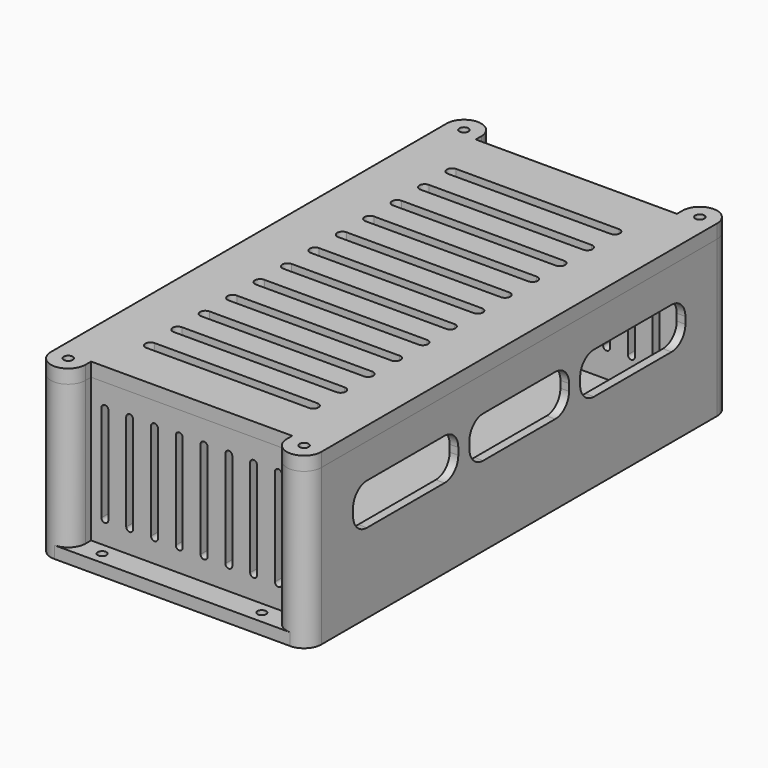
from build123d import *

# Parameters (mm, degrees)
F0_W      = 78.13
F0_H      = 138.9
F0_W_2    = 71.13
F0_H_2    = 131.9
F1_DEPTH  = 25
F2_W      = 71.13
F2_H      = 131.9
F3_DEPTH  = 2
F4_R      = 1.8
F5_DEPTH  = 6
F6_DEPTH  = 15
F7_DEPTH  = 5
F9_DEPTH  = 25
F11_DEPTH = 3.5
F12_W     = 73.13
F12_H     = 133.9
F12_W_2   = 71.13
F12_H_2   = 131.9
F13_DEPTH = 37
F14_W     = 56.34
F14_H     = 1
F14_W_2   = 1
F14_H_2   = 116.795
F14_H_3   = 107.2624295342
F15_DEPTH = 6
F17_DEPTH = 45
F19_DEPTH = 4
F20_W     = 72.53
F20_H     = 133.3
F21_DEPTH = 2
F23_DEPTH = 10
F24_R     = 1.3
F25_DEPTH = 20
F26_R     = 1.3
F27_DEPTH = 15
F28_W     = 68.13
F28_H     = 7
F29_DEPTH = 3.5
F30_R     = 1.25
F31_DEPTH = 25
F32_R     = 1.25
F33_DEPTH = 25
F35_DEPTH = 213


with BuildPart() as f1:
    # F0 (on Top) → F1 (new body)
    with BuildSketch(Plane.XY):
        with Locations((-1.6999974132, -1.6999974132)):
            Rectangle(F0_W, F0_H)
        with Locations((-1.6999974132, -1.6999974132)):
            Rectangle(F0_W_2, F0_H_2, mode=Mode.SUBTRACT)
    extrude(amount=F1_DEPTH)

    # F2 (on face) → F3 (join)
    with BuildSketch(Plane(origin=(0, 0, 0), x_dir=(1, 0, 0), z_dir=(0, 0, -1))):
        with Locations((-1.6999974132, 1.6999974132)):
            Rectangle(F2_W, F2_H)
    extrude(amount=-F3_DEPTH)

    # F4 (on face) → F5 (join)
    with BuildSketch(Plane.XY.offset(2)):
        with BuildLine():
            ThreePointArc((30.1700025868, -59.9299974132), (27.8294791411, -60.8994739674), (26.8600025868, -63.2399974132))
            Line((26.8600025868, -63.2399974132), (26.8600025868, -67.1499974132))
            Line((26.8600025868, -67.1499974132), (26.8600025868, -67.6499974132))
            Line((26.8600025868, -67.6499974132), (33.8650025868, -67.6499974132))
            Line((33.8650025868, -67.6499974132), (33.8650025868, -59.9299974132))
            Line((33.8650025868, -59.9299974132), (33.3000025868, -59.9299974132))
            Line((33.3000025868, -59.9299974132), (30.1700025868, -59.9299974132))
        make_face()
        with Locations((30.1700025868, -63.2399974132)):
            Circle(F4_R, mode=Mode.SUBTRACT)
        with BuildLine():
            ThreePointArc((-29.4799974132, -63.6399974132), (-30.566631255, -61.016631255), (-33.1899974132, -59.9299974132))
            Line((-33.1899974132, -59.9299974132), (-36.6999974132, -59.9299974132))
            Line((-36.6999974132, -59.9299974132), (-37.2649974132, -59.9299974132))
            Line((-37.2649974132, -59.9299974132), (-37.2649974132, -67.6499974132))
            Line((-37.2649974132, -67.6499974132), (-29.4799974132, -67.6499974132))
            Line((-29.4799974132, -67.6499974132), (-29.4799974132, -67.1499974132))
            Line((-29.4799974132, -67.1499974132), (-29.4799974132, -63.6399974132))
        make_face()
        with Locations((-33.1899974132, -63.6399974132)):
            Circle(F4_R, mode=Mode.SUBTRACT)
        with BuildLine():
            Line((-36.6999974132, 47.3750025868), (-33.6899974132, 47.3750025868))
            ThreePointArc((-33.6899974132, 47.3750025868), (-30.0649974132, 51.0000025868), (-33.6899974132, 54.6250025868))
            Line((-33.6899974132, 54.6250025868), (-36.6999974132, 54.6250025868))
            Line((-36.6999974132, 54.6250025868), (-37.2649974132, 54.6250025868))
            Line((-37.2649974132, 54.6250025868), (-37.2649974132, 47.3750025868))
            Line((-37.2649974132, 47.3750025868), (-36.6999974132, 47.3750025868))
        make_face()
        with Locations((-33.6899974132, 51.0000025868)):
            Circle(F4_R, mode=Mode.SUBTRACT)
        with BuildLine():
            Line((26.4150025868, 63.7500025868), (26.4150025868, 60.4900025868))
            ThreePointArc((26.4150025868, 60.4900025868), (27.476740505, 57.926740505), (30.0400025868, 56.8650025868))
            Line((30.0400025868, 56.8650025868), (33.8650025868, 56.8650025868))
            Line((33.8650025868, 56.8650025868), (33.8650025868, 64.2500025868))
            Line((33.8650025868, 64.2500025868), (26.4150025868, 64.2500025868))
            Line((26.4150025868, 64.2500025868), (26.4150025868, 63.7500025868))
        make_face()
        with BuildLine():
            ThreePointArc((30.0400025868, 58.6900025868), (28.7672103807, 61.762794793), (31.8400025868, 60.4900025868))
            ThreePointArc((31.8400025868, 60.4900025868), (31.312794793, 59.2172103807), (30.0400025868, 58.6900025868))
        make_face(mode=Mode.SUBTRACT)
    extrude(amount=F5_DEPTH)

    # F6 (add): a face of the model
    f6_faces = [f1.faces().sort_by_distance(p)[0] for p in [
        (35.7713430592, -1.6999974132, 25),
    ]]
    extrude(f6_faces, amount=F6_DEPTH)

    # F7 (add): a face of the model
    f7_faces = [f1.faces().sort_by_distance(p)[0] for p in [
        (35.7713430592, -1.6999974132, 40),
    ]]
    extrude(f7_faces, amount=F7_DEPTH)

    # F8 (on face) → F9 (cut)
    with BuildSketch(Plane.YZ.offset(37.3650025868)):
        with BuildLine():
            Line((11.3000025868, 35), (-1.6999974132, 35))
            Line((-1.6999974132, 35), (-14.6999974132, 35))
            ThreePointArc((-14.6999974132, 35), (-18.2355313191, 33.5355339059), (-19.6999974132, 30))
            Line((-19.6999974132, 30), (-19.6999974132, 28))
            ThreePointArc((-19.6999974132, 28), (-18.2355313191, 24.4644660941), (-14.6999974132, 23))
            Line((-14.6999974132, 23), (11.3000025868, 23))
            ThreePointArc((11.3000025868, 23), (14.8355364928, 24.4644660941), (16.3000025868, 28))
            Line((16.3000025868, 28), (16.3000025868, 30))
            ThreePointArc((16.3000025868, 30), (14.8355364928, 33.5355339059), (11.3000025868, 35))
        make_face()
        with BuildLine():
            Line((58.3000025868, 28), (58.3000025868, 30))
            ThreePointArc((58.3000025868, 30), (56.8355364928, 33.5355339059), (53.3000025868, 35))
            Line((53.3000025868, 35), (25.3000025868, 35))
            ThreePointArc((25.3000025868, 35), (21.7644686809, 33.5355339059), (20.3000025868, 30))
            Line((20.3000025868, 30), (20.3000025868, 28))
            ThreePointArc((20.3000025868, 28), (21.7644686809, 24.4644660941), (25.3000025868, 23))
            Line((25.3000025868, 23), (53.3000025868, 23))
            ThreePointArc((53.3000025868, 23), (56.8355364928, 24.4644660941), (58.3000025868, 28))
        make_face()
        with BuildLine():
            Line((-61.6999974132, 30), (-61.6999974132, 28))
            ThreePointArc((-61.6999974132, 28), (-60.2355313191, 24.4644660941), (-56.6999974132, 23))
            Line((-56.6999974132, 23), (-28.6999974132, 23))
            ThreePointArc((-28.6999974132, 23), (-25.1644635072, 24.4644660941), (-23.6999974132, 28))
            Line((-23.6999974132, 28), (-23.6999974132, 30))
            ThreePointArc((-23.6999974132, 30), (-25.1644635072, 33.5355339059), (-28.6999974132, 35))
            Line((-28.6999974132, 35), (-56.6999974132, 35))
            ThreePointArc((-56.6999974132, 35), (-60.2355313191, 33.5355339059), (-61.6999974132, 30))
        make_face()
    extrude(amount=-F9_DEPTH, mode=Mode.SUBTRACT)

    # F10 (on face) → F11 (cut, through all)
    with BuildSketch(Plane(origin=(-40.7649974132, 0, 0), x_dir=(0, -1, 0), z_dir=(-1, 0, 0))):
        with BuildLine():
            ThreePointArc((-59.6591697992, 39), (-60.0000025868, 39.03351143), (-60.3408353745, 39))
            Line((-60.3408353745, 39), (-59.6591697992, 39))
        make_face()
        with BuildLine():
            Line((-59.6591697992, 39), (-60.3408353745, 39))
            ThreePointArc((-60.3408353745, 39), (-61.3525848169, 38.3939263573), (-61.7500025868, 37.28351143))
            Line((-61.7500025868, 37.28351143), (-61.7500025868, 7.75))
            ThreePointArc((-61.7500025868, 7.75), (-60.0000025868, 6), (-58.2500025868, 7.75))
            Line((-58.2500025868, 7.75), (-58.2500025868, 37.28351143))
            ThreePointArc((-58.2500025868, 37.28351143), (-58.6474203567, 38.3939263573), (-59.6591697992, 39))
        make_face()
        with BuildLine():
            ThreePointArc((-46.6408353745, 39), (-47.6525848169, 38.3939263573), (-48.0500025868, 37.28351143))
            Line((-48.0500025868, 37.28351143), (-48.0500025868, 7.75))
            ThreePointArc((-48.0500025868, 7.75), (-46.3000025868, 6), (-44.5500025868, 7.75))
            Line((-44.5500025868, 7.75), (-44.5500025868, 37.28351143))
            ThreePointArc((-44.5500025868, 37.28351143), (-44.9474203567, 38.3939263573), (-45.9591697992, 39))
            Line((-45.9591697992, 39), (-46.6408353745, 39))
        make_face()
        with BuildLine():
            ThreePointArc((-45.9591697992, 39), (-46.3000025868, 39.03351143), (-46.6408353745, 39))
            Line((-46.6408353745, 39), (-45.9591697992, 39))
        make_face()
        with BuildLine():
            ThreePointArc((-32.9408353745, 39), (-33.9525848169, 38.3939263573), (-34.3500025868, 37.28351143))
            Line((-34.3500025868, 37.28351143), (-34.3500025868, 7.75))
            ThreePointArc((-34.3500025868, 7.75), (-32.6000025868, 6), (-30.8500025868, 7.75))
            Line((-30.8500025868, 7.75), (-30.8500025868, 37.28351143))
            ThreePointArc((-30.8500025868, 37.28351143), (-31.2474203567, 38.3939263573), (-32.2591697992, 39))
            Line((-32.2591697992, 39), (-32.9408353745, 39))
        make_face()
        with BuildLine():
            ThreePointArc((-32.2591697992, 39), (-32.6000025868, 39.03351143), (-32.9408353745, 39))
            Line((-32.9408353745, 39), (-32.2591697992, 39))
        make_face()
        with BuildLine():
            ThreePointArc((-19.2408353745, 39), (-20.2525848169, 38.3939263573), (-20.6500025868, 37.28351143))
            Line((-20.6500025868, 37.28351143), (-20.6500025868, 7.75))
            ThreePointArc((-20.6500025868, 7.75), (-18.9000025868, 6), (-17.1500025868, 7.75))
            Line((-17.1500025868, 7.75), (-17.1500025868, 37.28351143))
            ThreePointArc((-17.1500025868, 37.28351143), (-17.5474203567, 38.3939263573), (-18.5591697992, 39))
            Line((-18.5591697992, 39), (-19.2408353745, 39))
        make_face()
        with BuildLine():
            ThreePointArc((-18.5591697992, 39), (-18.9000025868, 39.03351143), (-19.2408353745, 39))
            Line((-19.2408353745, 39), (-18.5591697992, 39))
        make_face()
        with BuildLine():
            ThreePointArc((-5.5408353745, 39), (-6.5525848169, 38.3939263573), (-6.9500025868, 37.28351143))
            Line((-6.9500025868, 37.28351143), (-6.9500025868, 7.75))
            ThreePointArc((-6.9500025868, 7.75), (-5.2000025868, 6), (-3.4500025868, 7.75))
            Line((-3.4500025868, 7.75), (-3.4500025868, 37.28351143))
            ThreePointArc((-3.4500025868, 37.28351143), (-3.8474203567, 38.3939263573), (-4.8591697992, 39))
            Line((-4.8591697992, 39), (-5.5408353745, 39))
        make_face()
        with BuildLine():
            ThreePointArc((-4.8591697992, 39), (-5.2000025868, 39.03351143), (-5.5408353745, 39))
            Line((-5.5408353745, 39), (-4.8591697992, 39))
        make_face()
        with BuildLine():
            ThreePointArc((8.1591646255, 39), (7.1474151831, 38.3939263573), (6.7499974132, 37.28351143))
            Line((6.7499974132, 37.28351143), (6.7499974132, 7.75))
            ThreePointArc((6.7499974132, 7.75), (8.4999974132, 6), (10.2499974132, 7.75))
            Line((10.2499974132, 7.75), (10.2499974132, 37.28351143))
            ThreePointArc((10.2499974132, 37.28351143), (9.8525796433, 38.3939263573), (8.8408302008, 39))
            Line((8.8408302008, 39), (8.1591646255, 39))
        make_face()
        with BuildLine():
            ThreePointArc((8.8408302008, 39), (8.4999974132, 39.03351143), (8.1591646255, 39))
            Line((8.1591646255, 39), (8.8408302008, 39))
        make_face()
        with BuildLine():
            ThreePointArc((21.8591646255, 39), (20.8474151831, 38.3939263573), (20.4499974132, 37.28351143))
            Line((20.4499974132, 37.28351143), (20.4499974132, 7.75))
            ThreePointArc((20.4499974132, 7.75), (22.1999974132, 6), (23.9499974132, 7.75))
            Line((23.9499974132, 7.75), (23.9499974132, 37.28351143))
            ThreePointArc((23.9499974132, 37.28351143), (23.5525796433, 38.3939263573), (22.5408302008, 39))
            Line((22.5408302008, 39), (21.8591646255, 39))
        make_face()
        with BuildLine():
            ThreePointArc((22.5408302008, 39), (22.1999974132, 39.03351143), (21.8591646255, 39))
            Line((21.8591646255, 39), (22.5408302008, 39))
        make_face()
        with BuildLine():
            ThreePointArc((35.5591646255, 39), (34.5474151831, 38.3939263573), (34.1499974132, 37.28351143))
            Line((34.1499974132, 37.28351143), (34.1499974132, 7.75))
            ThreePointArc((34.1499974132, 7.75), (35.8999974132, 6), (37.6499974132, 7.75))
            Line((37.6499974132, 7.75), (37.6499974132, 37.28351143))
            ThreePointArc((37.6499974132, 37.28351143), (37.2525796433, 38.3939263573), (36.2408302008, 39))
            Line((36.2408302008, 39), (35.5591646255, 39))
        make_face()
        with BuildLine():
            ThreePointArc((36.2408302008, 39), (35.8999974132, 39.03351143), (35.5591646255, 39))
            Line((35.5591646255, 39), (36.2408302008, 39))
        make_face()
        with BuildLine():
            ThreePointArc((49.2591646255, 39), (48.2474151831, 38.3939263573), (47.8499974132, 37.28351143))
            Line((47.8499974132, 37.28351143), (47.8499974132, 7.75))
            ThreePointArc((47.8499974132, 7.75), (49.5999974132, 6), (51.3499974132, 7.75))
            Line((51.3499974132, 7.75), (51.3499974132, 37.28351143))
            ThreePointArc((51.3499974132, 37.28351143), (50.9525796433, 38.3939263573), (49.9408302008, 39))
            Line((49.9408302008, 39), (49.2591646255, 39))
        make_face()
        with BuildLine():
            ThreePointArc((49.9408302008, 39), (49.5999974132, 39.03351143), (49.2591646255, 39))
            Line((49.2591646255, 39), (49.9408302008, 39))
        make_face()
        with BuildLine():
            ThreePointArc((62.9591646255, 39), (61.9474151831, 38.3939263573), (61.5499974132, 37.28351143))
            Line((61.5499974132, 37.28351143), (61.5499974132, 7.75))
            ThreePointArc((61.5499974132, 7.75), (63.2999974132, 6), (65.0499974132, 7.75))
            Line((65.0499974132, 7.75), (65.0499974132, 37.28351143))
            ThreePointArc((65.0499974132, 37.28351143), (64.6525796433, 38.3939263573), (63.6408302008, 39))
            Line((63.6408302008, 39), (62.9591646255, 39))
        make_face()
        with BuildLine():
            ThreePointArc((63.6408302008, 39), (63.2999974132, 39.03351143), (62.9591646255, 39))
            Line((62.9591646255, 39), (63.6408302008, 39))
        make_face()
    extrude(amount=-F11_DEPTH, mode=Mode.SUBTRACT)

    # F12 (on face) → F13 (cut, through all)
    with BuildSketch(Plane.XY.offset(45)):
        with Locations((-1.6999974132, -1.6999974132)):
            Rectangle(F12_W, F12_H)
        with Locations((-1.6999974132, -1.6999974132)):
            Rectangle(F12_W_2, F12_H_2, mode=Mode.SUBTRACT)
    extrude(amount=-F13_DEPTH, mode=Mode.SUBTRACT)

    # F14 (on face) → F15 (cut, through all)
    with BuildSketch(Plane.XY.offset(8)):
        Polygon((26.4150025868, 65.2500025868), (-38.2649974132, 65.2500025868), (-38.2649974132, 54.6365268528), (-37.2649974132, 54.6365268528), (-37.2649974132, 64.2500025868), (26.4150025868, 64.2500025868), align=None)
        with Locations((-1.3099974132, -68.1499974132)):
            Rectangle(F14_W, F14_H)
        with Locations((34.3650025868, -1.5324974132)):
            Rectangle(F14_W_2, F14_H_2)
        with Locations((-37.7649974132, -6.2987826461)):
            Rectangle(F14_W_2, F14_H_3)
    extrude(amount=-F15_DEPTH, mode=Mode.SUBTRACT)

    # F16 (on face) → F17 (join, through all)
    with BuildSketch(Plane.XY.offset(45)):
        with BuildLine():
            Line((-40.7649974132, 69.7500025868), (-40.7649974132, 67.7500025868))
            Line((-40.7649974132, 67.7500025868), (-30.7649974132, 67.7500025868))
            Line((-30.7649974132, 67.7500025868), (-30.7649974132, 69.7500025868))
            ThreePointArc((-30.7649974132, 69.7500025868), (-35.7649974132, 74.7500025868), (-40.7649974132, 69.7500025868))
        make_face()
        with BuildLine():
            Line((27.3650025868, 67.7500025868), (37.3650025868, 67.7500025868))
            Line((37.3650025868, 67.7500025868), (37.3650025868, 69.7500025868))
            ThreePointArc((37.3650025868, 69.7500025868), (32.3650025868, 74.7500025868), (27.3650025868, 69.7500025868))
            Line((27.3650025868, 69.7500025868), (27.3650025868, 67.7500025868))
        make_face()
        with BuildLine():
            Line((-30.7649974132, -71.1499974132), (-40.7649974132, -71.1499974132))
            Line((-40.7649974132, -71.1499974132), (-40.7649974132, -73.1499974132))
            ThreePointArc((-40.7649974132, -73.1499974132), (-35.7649974132, -78.1499974132), (-30.7649974132, -73.1499974132))
            Line((-30.7649974132, -73.1499974132), (-30.7649974132, -71.1499974132))
        make_face()
        with BuildLine():
            Line((37.3650025868, -73.1499974132), (37.3650025868, -71.1499974132))
            Line((37.3650025868, -71.1499974132), (27.3650025868, -71.1499974132))
            Line((27.3650025868, -71.1499974132), (27.3650025868, -73.1499974132))
            ThreePointArc((27.3650025868, -73.1499974132), (32.3650025868, -78.1499974132), (37.3650025868, -73.1499974132))
        make_face()
    extrude(amount=-F17_DEPTH)

    # F26 (on face) → F27 (cut)
    with BuildSketch(Plane.XY.offset(45)):
        with Locations((-35.7649974132, 69.7500025868)):
            Circle(F26_R)
        with Locations((32.3650025868, 69.7500025868)):
            Circle(F26_R)
        with Locations((32.3650025868, -73.1499974132)):
            Circle(F26_R)
        with Locations((-35.7649974132, -73.1499974132)):
            Circle(F26_R)
    extrude(amount=-F27_DEPTH, mode=Mode.SUBTRACT)

    # F28 (on face) → F29 (join)
    with BuildSketch(Plane(origin=(0, 0, 0), x_dir=(1, 0, 0), z_dir=(0, 0, -1))):
        with Locations((-1.6999974132, 74.6499974132)):
            Rectangle(F28_W, F28_H)
        with Locations((-1.6999974132, -71.2500025868)):
            Rectangle(F28_W, F28_H)
    extrude(amount=-F29_DEPTH)

    # F30 (on face) → F31 (cut)
    with BuildSketch(Plane.XY.offset(3.5)):
        with BuildLine():
            ThreePointArc((-26.0149974132, 71.2500025868), (-24.7649974132, 70.0000025868), (-23.5149974132, 71.2500025868))
            ThreePointArc((-23.5149974132, 71.2500025868), (-24.7649974132, 72.5000025868), (-26.0149974132, 71.2500025868))
        make_face()
        with Locations((21.3650025868, 71.2500025868)):
            Circle(F30_R)
    extrude(amount=-F31_DEPTH, mode=Mode.SUBTRACT)

    # F32 (on face) → F33 (cut)
    with BuildSketch(Plane.XY.offset(3.5)):
        with Locations((21.3650025868, -74.6499974132)):
            Circle(F32_R)
        with BuildLine():
            ThreePointArc((-26.0149974132, -74.6499974132), (-24.7649974132, -75.8999974132), (-23.5149974132, -74.6499974132))
            ThreePointArc((-23.5149974132, -74.6499974132), (-24.7649974132, -73.3999974132), (-26.0149974132, -74.6499974132))
        make_face()
    extrude(amount=-F33_DEPTH, mode=Mode.SUBTRACT)

    # F34 (on face) → F35 (cut)
    with BuildSketch(Plane.XZ.offset(71.1499974132)):
        with BuildLine():
            Line((-27.7649974132, 38.25), (-27.7649974132, 24.25))
            Line((-27.7649974132, 24.25), (-27.7649974132, 10.25))
            ThreePointArc((-27.7649974132, 10.25), (-26.7649974132, 9.25), (-25.7649974132, 10.25))
            Line((-25.7649974132, 10.25), (-25.7649974132, 38.25))
            ThreePointArc((-25.7649974132, 38.25), (-26.7649974132, 39.25), (-27.7649974132, 38.25))
        make_face()
        with BuildLine():
            Line((-18.6049974132, 10.25), (-18.6049974132, 38.25))
            ThreePointArc((-18.6049974132, 38.25), (-19.6049974132, 39.25), (-20.6049974132, 38.25))
            Line((-20.6049974132, 38.25), (-20.6049974132, 24.25))
            Line((-20.6049974132, 24.25), (-20.6049974132, 10.25))
            ThreePointArc((-20.6049974132, 10.25), (-19.6049974132, 9.25), (-18.6049974132, 10.25))
        make_face()
        with BuildLine():
            Line((-11.4449974132, 10.25), (-11.4449974132, 38.25))
            ThreePointArc((-11.4449974132, 38.25), (-12.4449974132, 39.25), (-13.4449974132, 38.25))
            Line((-13.4449974132, 38.25), (-13.4449974132, 24.25))
            Line((-13.4449974132, 24.25), (-13.4449974132, 10.25))
            ThreePointArc((-13.4449974132, 10.25), (-12.4449974132, 9.25), (-11.4449974132, 10.25))
        make_face()
        with BuildLine():
            Line((-4.2849974132, 10.25), (-4.2849974132, 38.25))
            ThreePointArc((-4.2849974132, 38.25), (-5.2849974132, 39.25), (-6.2849974132, 38.25))
            Line((-6.2849974132, 38.25), (-6.2849974132, 24.25))
            Line((-6.2849974132, 24.25), (-6.2849974132, 10.25))
            ThreePointArc((-6.2849974132, 10.25), (-5.2849974132, 9.25), (-4.2849974132, 10.25))
        make_face()
        with BuildLine():
            Line((2.8750025868, 10.25), (2.8750025868, 38.25))
            ThreePointArc((2.8750025868, 38.25), (1.8750025868, 39.25), (0.8750025868, 38.25))
            Line((0.8750025868, 38.25), (0.8750025868, 24.25))
            Line((0.8750025868, 24.25), (0.8750025868, 10.25))
            ThreePointArc((0.8750025868, 10.25), (1.8750025868, 9.25), (2.8750025868, 10.25))
        make_face()
        with BuildLine():
            Line((10.0350025868, 10.25), (10.0350025868, 38.25))
            ThreePointArc((10.0350025868, 38.25), (9.0350025868, 39.25), (8.0350025868, 38.25))
            Line((8.0350025868, 38.25), (8.0350025868, 24.25))
            Line((8.0350025868, 24.25), (8.0350025868, 10.25))
            ThreePointArc((8.0350025868, 10.25), (9.0350025868, 9.25), (10.0350025868, 10.25))
        make_face()
        with BuildLine():
            Line((17.1950025868, 10.25), (17.1950025868, 38.25))
            ThreePointArc((17.1950025868, 38.25), (16.1950025868, 39.25), (15.1950025868, 38.25))
            Line((15.1950025868, 38.25), (15.1950025868, 24.25))
            Line((15.1950025868, 24.25), (15.1950025868, 10.25))
            ThreePointArc((15.1950025868, 10.25), (16.1950025868, 9.25), (17.1950025868, 10.25))
        make_face()
        with BuildLine():
            Line((24.3550025868, 10.25), (24.3550025868, 38.25))
            ThreePointArc((24.3550025868, 38.25), (23.3550025868, 39.25), (22.3550025868, 38.25))
            Line((22.3550025868, 38.25), (22.3550025868, 24.25))
            Line((22.3550025868, 24.25), (22.3550025868, 10.25))
            ThreePointArc((22.3550025868, 10.25), (23.3550025868, 9.25), (24.3550025868, 10.25))
        make_face()
    extrude(amount=-F35_DEPTH, mode=Mode.SUBTRACT)


with BuildPart() as f19:
    # F18 (on face) → F19 (new body)
    with BuildSketch(Plane.XY.offset(45)):
        with BuildLine():
            Line((27.3650025868, 67.7500025868), (-30.7649974132, 67.7500025868))
            Line((-30.7649974132, 67.7500025868), (-30.7649974132, 69.7500025868))
            ThreePointArc((-30.7649974132, 69.7500025868), (-35.7649974132, 74.7500025868), (-40.7649974132, 69.7500025868))
            Line((-40.7649974132, 69.7500025868), (-40.7649974132, -73.1499974132))
            ThreePointArc((-40.7649974132, -73.1499974132), (-35.7649974132, -78.1499974132), (-30.7649974132, -73.1499974132))
            Line((-30.7649974132, -73.1499974132), (-30.7649974132, -71.1499974132))
            Line((-30.7649974132, -71.1499974132), (27.3650025868, -71.1499974132))
            Line((27.3650025868, -71.1499974132), (27.3650025868, -73.1499974132))
            ThreePointArc((27.3650025868, -73.1499974132), (32.3650025868, -78.1499974132), (37.3650025868, -73.1499974132))
            Line((37.3650025868, -73.1499974132), (37.3650025868, 69.7500025868))
            ThreePointArc((37.3650025868, 69.7500025868), (32.3650025868, 74.7500025868), (27.3650025868, 69.7500025868))
            Line((27.3650025868, 69.7500025868), (27.3650025868, 67.7500025868))
        make_face()
    extrude(amount=F19_DEPTH)

    # F20 (on face) → F21 (join)
    with BuildSketch(Plane(origin=(0, 0, 45), x_dir=(1, 0, 0), z_dir=(0, 0, -1))):
        with Locations((-1.6999974132, 1.6999974132)):
            Rectangle(F20_W, F20_H)
    extrude(amount=F21_DEPTH)

    # F22 (on face) → F23 (cut)
    with BuildSketch(Plane.XY.offset(49)):
        with BuildLine():
            Line((-25.1999974132, -58.1499974132), (-1.6999974132, -58.1499974132))
            Line((-1.6999974132, -58.1499974132), (21.8000025868, -58.1499974132))
            ThreePointArc((21.8000025868, -58.1499974132), (23.3000025868, -56.6499974132), (21.8000025868, -55.1499974132))
            Line((21.8000025868, -55.1499974132), (-25.1999974132, -55.1499974132))
            ThreePointArc((-25.1999974132, -55.1499974132), (-26.6999974132, -56.6499974132), (-25.1999974132, -58.1499974132))
        make_face()
        with BuildLine():
            ThreePointArc((21.8000025868, -48.2499974132), (23.3000025868, -46.7499974132), (21.8000025868, -45.2499974132))
            Line((21.8000025868, -45.2499974132), (-25.1999974132, -45.2499974132))
            ThreePointArc((-25.1999974132, -45.2499974132), (-26.6999974132, -46.7499974132), (-25.1999974132, -48.2499974132))
            Line((-25.1999974132, -48.2499974132), (-1.6999974132, -48.2499974132))
            Line((-1.6999974132, -48.2499974132), (21.8000025868, -48.2499974132))
        make_face()
        with BuildLine():
            ThreePointArc((21.8000025868, -38.3499974132), (23.3000025868, -36.8499974132), (21.8000025868, -35.3499974132))
            Line((21.8000025868, -35.3499974132), (-25.1999974132, -35.3499974132))
            ThreePointArc((-25.1999974132, -35.3499974132), (-26.6999974132, -36.8499974132), (-25.1999974132, -38.3499974132))
            Line((-25.1999974132, -38.3499974132), (-1.6999974132, -38.3499974132))
            Line((-1.6999974132, -38.3499974132), (21.8000025868, -38.3499974132))
        make_face()
        with BuildLine():
            ThreePointArc((21.8000025868, -28.4499974132), (23.3000025868, -26.9499974132), (21.8000025868, -25.4499974132))
            Line((21.8000025868, -25.4499974132), (-25.1999974132, -25.4499974132))
            ThreePointArc((-25.1999974132, -25.4499974132), (-26.6999974132, -26.9499974132), (-25.1999974132, -28.4499974132))
            Line((-25.1999974132, -28.4499974132), (-1.6999974132, -28.4499974132))
            Line((-1.6999974132, -28.4499974132), (21.8000025868, -28.4499974132))
        make_face()
        with BuildLine():
            ThreePointArc((21.8000025868, -18.5499974132), (23.3000025868, -17.0499974132), (21.8000025868, -15.5499974132))
            Line((21.8000025868, -15.5499974132), (-25.1999974132, -15.5499974132))
            ThreePointArc((-25.1999974132, -15.5499974132), (-26.6999974132, -17.0499974132), (-25.1999974132, -18.5499974132))
            Line((-25.1999974132, -18.5499974132), (-1.6999974132, -18.5499974132))
            Line((-1.6999974132, -18.5499974132), (21.8000025868, -18.5499974132))
        make_face()
        with BuildLine():
            ThreePointArc((21.8000025868, -8.6499974132), (23.3000025868, -7.1499974132), (21.8000025868, -5.6499974132))
            Line((21.8000025868, -5.6499974132), (-25.1999974132, -5.6499974132))
            ThreePointArc((-25.1999974132, -5.6499974132), (-26.6999974132, -7.1499974132), (-25.1999974132, -8.6499974132))
            Line((-25.1999974132, -8.6499974132), (-1.6999974132, -8.6499974132))
            Line((-1.6999974132, -8.6499974132), (21.8000025868, -8.6499974132))
        make_face()
        with BuildLine():
            ThreePointArc((21.8000025868, 1.2500025868), (23.3000025868, 2.7500025868), (21.8000025868, 4.2500025868))
            Line((21.8000025868, 4.2500025868), (-25.1999974132, 4.2500025868))
            ThreePointArc((-25.1999974132, 4.2500025868), (-26.6999974132, 2.7500025868), (-25.1999974132, 1.2500025868))
            Line((-25.1999974132, 1.2500025868), (-1.6999974132, 1.2500025868))
            Line((-1.6999974132, 1.2500025868), (21.8000025868, 1.2500025868))
        make_face()
        with BuildLine():
            ThreePointArc((21.8000025868, 11.1500025868), (23.3000025868, 12.6500025868), (21.8000025868, 14.1500025868))
            Line((21.8000025868, 14.1500025868), (-25.1999974132, 14.1500025868))
            ThreePointArc((-25.1999974132, 14.1500025868), (-26.6999974132, 12.6500025868), (-25.1999974132, 11.1500025868))
            Line((-25.1999974132, 11.1500025868), (-1.6999974132, 11.1500025868))
            Line((-1.6999974132, 11.1500025868), (21.8000025868, 11.1500025868))
        make_face()
        with BuildLine():
            ThreePointArc((21.8000025868, 21.0500025868), (23.3000025868, 22.5500025868), (21.8000025868, 24.0500025868))
            Line((21.8000025868, 24.0500025868), (-25.1999974132, 24.0500025868))
            ThreePointArc((-25.1999974132, 24.0500025868), (-26.6999974132, 22.5500025868), (-25.1999974132, 21.0500025868))
            Line((-25.1999974132, 21.0500025868), (-1.6999974132, 21.0500025868))
            Line((-1.6999974132, 21.0500025868), (21.8000025868, 21.0500025868))
        make_face()
        with BuildLine():
            ThreePointArc((21.8000025868, 30.9500025868), (23.3000025868, 32.4500025868), (21.8000025868, 33.9500025868))
            Line((21.8000025868, 33.9500025868), (-25.1999974132, 33.9500025868))
            ThreePointArc((-25.1999974132, 33.9500025868), (-26.6999974132, 32.4500025868), (-25.1999974132, 30.9500025868))
            Line((-25.1999974132, 30.9500025868), (-1.6999974132, 30.9500025868))
            Line((-1.6999974132, 30.9500025868), (21.8000025868, 30.9500025868))
        make_face()
        with BuildLine():
            ThreePointArc((21.8000025868, 40.8500025868), (23.3000025868, 42.3500025868), (21.8000025868, 43.8500025868))
            Line((21.8000025868, 43.8500025868), (-25.1999974132, 43.8500025868))
            ThreePointArc((-25.1999974132, 43.8500025868), (-26.6999974132, 42.3500025868), (-25.1999974132, 40.8500025868))
            Line((-25.1999974132, 40.8500025868), (-1.6999974132, 40.8500025868))
            Line((-1.6999974132, 40.8500025868), (21.8000025868, 40.8500025868))
        make_face()
        with BuildLine():
            ThreePointArc((21.8000025868, 50.7500025868), (23.3000025868, 52.2500025868), (21.8000025868, 53.7500025868))
            Line((21.8000025868, 53.7500025868), (-25.1999974132, 53.7500025868))
            ThreePointArc((-25.1999974132, 53.7500025868), (-26.6999974132, 52.2500025868), (-25.1999974132, 50.7500025868))
            Line((-25.1999974132, 50.7500025868), (-1.6999974132, 50.7500025868))
            Line((-1.6999974132, 50.7500025868), (21.8000025868, 50.7500025868))
        make_face()
    extrude(amount=-F23_DEPTH, mode=Mode.SUBTRACT)

    # F24 (on face) → F25 (cut)
    with BuildSketch(Plane.XY.offset(49)):
        with Locations((-35.7649974132, 69.7500025868)):
            Circle(F24_R)
        with Locations((32.3650025868, 69.7500025868)):
            Circle(F24_R)
        with Locations((-35.7649974132, -73.1499974132)):
            Circle(F24_R)
        with Locations((32.3650025868, -73.1499974132)):
            Circle(F24_R)
    extrude(amount=-F25_DEPTH, mode=Mode.SUBTRACT)


solid = Compound([f1.part, f19.part])
